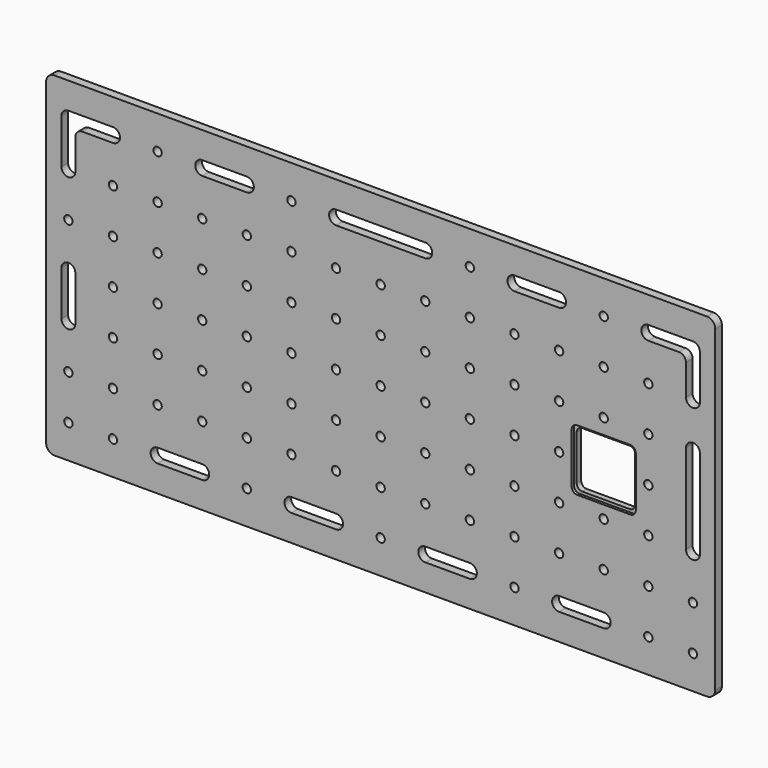
from build123d import *

# Parameters (mm, degrees)
F1_DEPTH = 19.05
F3_DEPTH = 6.35
F2_R     = 9.525
F4_DEPTH = 19.05
F5_DEPTH = 19.05


# Not quite as in the source:
# - a feature names something its author has since deleted; it is built from what else it names


with BuildPart() as f1:
    # F0 (on Front) → F1 (new body)
    with BuildSketch(Plane.XZ):
        with BuildLine():
            ThreePointArc((762, 361.95), (756.4203841816, 375.4203841816), (742.95, 381))
            Line((742.95, 381), (-742.95, 381))
            ThreePointArc((-742.95, 381), (-756.4203841816, 375.4203841816), (-762, 361.95))
            Line((-762, 361.95), (-762, -361.95))
            ThreePointArc((-762, -361.95), (-756.4203841816, -375.4203841816), (-742.95, -381))
            Line((-742.95, -381), (742.95, -381))
            ThreePointArc((742.95, -381), (756.4203841816, -375.4203841816), (762, -361.95))
            Line((762, -361.95), (762, 361.95))
        make_face()
    extrude(amount=F1_DEPTH)

    # F2 (on face) → F3 (cut)
    with BuildSketch(Plane.XZ.offset(19.05)):
        with BuildLine():
            ThreePointArc((435.0450174809, -60.2549825191), (438.7647613598, -69.2352386402), (447.7450174809, -72.9549825191))
            Line((447.7450174809, -72.9549825191), (568.3950174809, -72.9549825191))
            ThreePointArc((568.3950174809, -72.9549825191), (577.3752736019, -69.2352386402), (581.0950174809, -60.2549825191))
            Line((581.0950174809, -60.2549825191), (581.0950174809, 54.0450174809))
            ThreePointArc((581.0950174809, 54.0450174809), (577.3752736019, 63.0252736019), (568.3950174809, 66.7450174809))
            Line((568.3950174809, 66.7450174809), (447.7450174809, 66.7450174809))
            ThreePointArc((447.7450174809, 66.7450174809), (438.7647613598, 63.0252736019), (435.0450174809, 54.0450174809))
            Line((435.0450174809, 54.0450174809), (435.0450174809, -60.2549825191))
        make_face()
        with BuildLine():
            ThreePointArc((441.3950174809, 47.6950174809), (445.1147613598, 56.6752736019), (454.0950174809, 60.3950174809))
            Line((454.0950174809, 60.3950174809), (562.0450174809, 60.3950174809))
            ThreePointArc((562.0450174809, 60.3950174809), (571.0252736019, 56.6752736019), (574.7450174809, 47.6950174809))
            Line((574.7450174809, 47.6950174809), (574.7450174809, -53.9049825191))
            ThreePointArc((574.7450174809, -53.9049825191), (571.0252736019, -62.8852386402), (562.0450174809, -66.6049825191))
            Line((562.0450174809, -66.6049825191), (454.0950174809, -66.6049825191))
            ThreePointArc((454.0950174809, -66.6049825191), (445.1147613598, -62.8852386402), (441.3950174809, -53.9049825191))
            Line((441.3950174809, -53.9049825191), (441.3950174809, 47.6950174809))
        make_face(mode=Mode.SUBTRACT)
        with BuildLine():
            Line((562.0450174809, 60.3950174809), (454.0950174809, 60.3950174809))
            ThreePointArc((454.0950174809, 60.3950174809), (445.1147613598, 56.6752736019), (441.3950174809, 47.6950174809))
            Line((441.3950174809, 47.6950174809), (441.3950174809, -53.9049825191))
            ThreePointArc((441.3950174809, -53.9049825191), (445.1147613598, -62.8852386402), (454.0950174809, -66.6049825191))
            Line((454.0950174809, -66.6049825191), (562.0450174809, -66.6049825191))
            ThreePointArc((562.0450174809, -66.6049825191), (571.0252736019, -62.8852386402), (574.7450174809, -53.9049825191))
            Line((574.7450174809, -53.9049825191), (574.7450174809, 47.6950174809))
            ThreePointArc((574.7450174809, 47.6950174809), (571.0252736019, 56.6752736019), (562.0450174809, 60.3950174809))
        make_face()
    extrude(amount=-F3_DEPTH, mode=Mode.SUBTRACT)

    # F2 (on face) → F4 (cut)
    with BuildSketch(Plane.XZ.offset(19.05)):
        with Locations((711.2, -304.8)):
            Circle(F2_R)
        with Locations((711.2, -203.2)):
            Circle(F2_R)
        with Locations((609.6, -304.8)):
            Circle(F2_R)
        with Locations((609.6, -203.2)):
            Circle(F2_R)
        with Locations((609.6, -101.6)):
            Circle(F2_R)
        with Locations((609.6, 0)):
            Circle(F2_R)
        with Locations((609.6, 101.6)):
            Circle(F2_R)
        with Locations((609.6, 203.2)):
            Circle(F2_R)
        with Locations((508, -203.2)):
            Circle(F2_R)
        with Locations((508, -101.6)):
            Circle(F2_R)
        with Locations((508, 101.6)):
            Circle(F2_R)
        with Locations((508, 203.2)):
            Circle(F2_R)
        with Locations((508, 304.8)):
            Circle(F2_R)
        with Locations((406.4, -203.2)):
            Circle(F2_R)
        with Locations((406.4, -101.6)):
            Circle(F2_R)
        with Locations((406.4, 0)):
            Circle(F2_R)
        with Locations((406.4, 101.6)):
            Circle(F2_R)
        with Locations((406.4, 203.2)):
            Circle(F2_R)
        with Locations((304.8, -304.8)):
            Circle(F2_R)
        with Locations((304.8, -203.2)):
            Circle(F2_R)
        with Locations((304.8, -101.6)):
            Circle(F2_R)
        with Locations((304.8, 0)):
            Circle(F2_R)
        with Locations((304.8, 101.6)):
            Circle(F2_R)
        with Locations((304.8, 203.2)):
            Circle(F2_R)
        with Locations((203.2, -203.2)):
            Circle(F2_R)
        with Locations((203.2, -101.6)):
            Circle(F2_R)
        with Locations((203.2, 0)):
            Circle(F2_R)
        with Locations((203.2, 101.6)):
            Circle(F2_R)
        with Locations((203.2, 203.2)):
            Circle(F2_R)
        with Locations((203.2, 304.8)):
            Circle(F2_R)
        with Locations((101.6, -203.2)):
            Circle(F2_R)
        with Locations((101.6, -101.6)):
            Circle(F2_R)
        with Locations((101.6, 0)):
            Circle(F2_R)
        with Locations((101.6, 101.6)):
            Circle(F2_R)
        with Locations((101.6, 203.2)):
            Circle(F2_R)
        with Locations((0, -304.8)):
            Circle(F2_R)
        with Locations((0, -203.2)):
            Circle(F2_R)
        with Locations((0, -101.6)):
            Circle(F2_R)
        Circle(F2_R)
        with Locations((0, 101.6)):
            Circle(F2_R)
        with Locations((0, 203.2)):
            Circle(F2_R)
        with Locations((-101.6, -203.2)):
            Circle(F2_R)
        with Locations((-101.6, -101.6)):
            Circle(F2_R)
        with Locations((-101.6, 0)):
            Circle(F2_R)
        with Locations((-101.6, 101.6)):
            Circle(F2_R)
        with Locations((-101.6, 203.2)):
            Circle(F2_R)
        with Locations((-203.2, -203.2)):
            Circle(F2_R)
        with Locations((-203.2, -101.6)):
            Circle(F2_R)
        with Locations((-203.2, 0)):
            Circle(F2_R)
        with Locations((-203.2, 101.6)):
            Circle(F2_R)
        with Locations((-203.2, 203.2)):
            Circle(F2_R)
        with Locations((-203.2, 304.8)):
            Circle(F2_R)
        with Locations((-304.8, -304.8)):
            Circle(F2_R)
        with Locations((-304.8, -203.2)):
            Circle(F2_R)
        with Locations((-304.8, -101.6)):
            Circle(F2_R)
        with Locations((-304.8, 0)):
            Circle(F2_R)
        with Locations((-304.8, 101.6)):
            Circle(F2_R)
        with Locations((-304.8, 203.2)):
            Circle(F2_R)
        with Locations((-406.4, -203.2)):
            Circle(F2_R)
        with Locations((-406.4, -101.6)):
            Circle(F2_R)
        with Locations((-406.4, 0)):
            Circle(F2_R)
        with Locations((-406.4, 101.6)):
            Circle(F2_R)
        with Locations((-406.4, 203.2)):
            Circle(F2_R)
        with Locations((-508, -203.2)):
            Circle(F2_R)
        with Locations((-508, -101.6)):
            Circle(F2_R)
        with Locations((-508, 0)):
            Circle(F2_R)
        with Locations((-508, 101.6)):
            Circle(F2_R)
        with Locations((-508, 203.2)):
            Circle(F2_R)
        with Locations((-508, 304.8)):
            Circle(F2_R)
        with Locations((-609.6, -304.8)):
            Circle(F2_R)
        with Locations((-609.6, -203.2)):
            Circle(F2_R)
        with Locations((-609.6, -101.6)):
            Circle(F2_R)
        with Locations((-609.6, 0)):
            Circle(F2_R)
        with Locations((-609.6, 101.6)):
            Circle(F2_R)
        with Locations((-609.6, 203.2)):
            Circle(F2_R)
        with Locations((-711.2, -304.8)):
            Circle(F2_R)
        with Locations((-711.2, -203.2)):
            Circle(F2_R)
        with Locations((-711.2, 101.6)):
            Circle(F2_R)
        with BuildLine():
            Line((562.0450174809, 60.3950174809), (454.0950174809, 60.3950174809))
            ThreePointArc((454.0950174809, 60.3950174809), (445.1147613598, 56.6752736019), (441.3950174809, 47.6950174809))
            Line((441.3950174809, 47.6950174809), (441.3950174809, -53.9049825191))
            ThreePointArc((441.3950174809, -53.9049825191), (445.1147613598, -62.8852386402), (454.0950174809, -66.6049825191))
            Line((454.0950174809, -66.6049825191), (562.0450174809, -66.6049825191))
            ThreePointArc((562.0450174809, -66.6049825191), (571.0252736019, -62.8852386402), (574.7450174809, -53.9049825191))
            Line((574.7450174809, -53.9049825191), (574.7450174809, 47.6950174809))
            ThreePointArc((574.7450174809, 47.6950174809), (571.0252736019, 56.6752736019), (562.0450174809, 60.3950174809))
        make_face()
    extrude(amount=-F4_DEPTH, mode=Mode.SUBTRACT)

    # F2 (on face) → F5 (cut)
    with BuildSketch(Plane.XZ.offset(19.05)):
        with BuildLine():
            Line((-406.4, -288.925), (-508, -288.925))
            ThreePointArc((-508, -288.925), (-523.875, -304.8), (-508, -320.675))
            Line((-508, -320.675), (-406.4, -320.675))
            ThreePointArc((-406.4, -320.675), (-390.525, -304.8), (-406.4, -288.925))
        make_face()
        with BuildLine():
            Line((-101.6, -288.925), (-203.2, -288.925))
            ThreePointArc((-203.2, -288.925), (-219.075, -304.8), (-203.2, -320.675))
            Line((-203.2, -320.675), (-101.6, -320.675))
            ThreePointArc((-101.6, -320.675), (-85.725, -304.8), (-101.6, -288.925))
        make_face()
        with BuildLine():
            Line((203.2, -288.925), (101.6, -288.925))
            ThreePointArc((101.6, -288.925), (85.725, -304.8), (101.6, -320.675))
            Line((101.6, -320.675), (203.2, -320.675))
            ThreePointArc((203.2, -320.675), (219.075, -304.8), (203.2, -288.925))
        make_face()
        with BuildLine():
            Line((406.4, -320.675), (508, -320.675))
            ThreePointArc((508, -320.675), (523.875, -304.8), (508, -288.925))
            Line((508, -288.925), (406.4, -288.925))
            ThreePointArc((406.4, -288.925), (390.525, -304.8), (406.4, -320.675))
        make_face()
        with BuildLine():
            Line((727.075, -101.6), (727.075, 101.6))
            ThreePointArc((727.075, 101.6), (711.2, 117.475), (695.325, 101.6))
            Line((695.325, 101.6), (695.325, -101.6))
            ThreePointArc((695.325, -101.6), (711.2, -117.475), (727.075, -101.6))
        make_face()
        with BuildLine():
            Line((711.2, 320.675), (609.6, 320.675))
            ThreePointArc((609.6, 320.675), (593.725, 304.8), (609.6, 288.925))
            Line((609.6, 288.925), (679.45, 288.925))
            ThreePointArc((679.45, 288.925), (690.6753201513, 284.2753201513), (695.325, 273.05))
            Line((695.325, 273.05), (695.325, 203.2))
            ThreePointArc((695.325, 203.2), (711.2, 187.325), (727.075, 203.2))
            Line((727.075, 203.2), (727.075, 304.8))
            ThreePointArc((727.075, 304.8), (722.4253201513, 316.0253201513), (711.2, 320.675))
        make_face()
        with BuildLine():
            Line((406.4, 320.675), (304.8, 320.675))
            ThreePointArc((304.8, 320.675), (288.925, 304.8), (304.8, 288.925))
            Line((304.8, 288.925), (406.4, 288.925))
            ThreePointArc((406.4, 288.925), (422.275, 304.8), (406.4, 320.675))
        make_face()
        with BuildLine():
            Line((101.6, 320.675), (-101.6, 320.675))
            ThreePointArc((-101.6, 320.675), (-117.475, 304.8), (-101.6, 288.925))
            Line((-101.6, 288.925), (101.6, 288.925))
            ThreePointArc((101.6, 288.925), (117.475, 304.8), (101.6, 320.675))
        make_face()
        with BuildLine():
            Line((-304.8, 320.675), (-406.4, 320.675))
            ThreePointArc((-406.4, 320.675), (-422.275, 304.8), (-406.4, 288.925))
            Line((-406.4, 288.925), (-304.8, 288.925))
            ThreePointArc((-304.8, 288.925), (-288.925, 304.8), (-304.8, 320.675))
        make_face()
        with BuildLine():
            Line((-727.075, 304.8), (-727.075, 203.2))
            ThreePointArc((-727.075, 203.2), (-711.2, 187.325), (-695.325, 203.2))
            Line((-695.325, 203.2), (-695.325, 273.0499999853))
            ThreePointArc((-695.325, 273.0499999853), (-690.6753201487, 284.2753201392), (-679.4499999926, 288.9249999853))
            Line((-679.4499999926, 288.9249999853), (-609.6000000078, 288.9249999529))
            ThreePointArc((-609.6000000078, 288.9249999529), (-593.7250000006, 304.8000631767), (-609.6001264554, 320.6749999524))
            Line((-609.6001264554, 320.6749999524), (-711.0398251834, 320.6741919173))
            ThreePointArc((-711.0398251834, 320.6741919173), (-722.3685462301, 316.0818083704), (-727.075, 304.8))
        make_face()
        with BuildLine():
            Line((-727.075, 0), (-727.075, -101.6))
            ThreePointArc((-727.075, -101.6), (-711.2, -117.475), (-695.325, -101.6))
            Line((-695.325, -101.6), (-695.325, 0))
            ThreePointArc((-695.325, 0), (-711.2, 15.875), (-727.075, 0))
        make_face()
    extrude(amount=-F5_DEPTH, mode=Mode.SUBTRACT)


solid = f1.part
